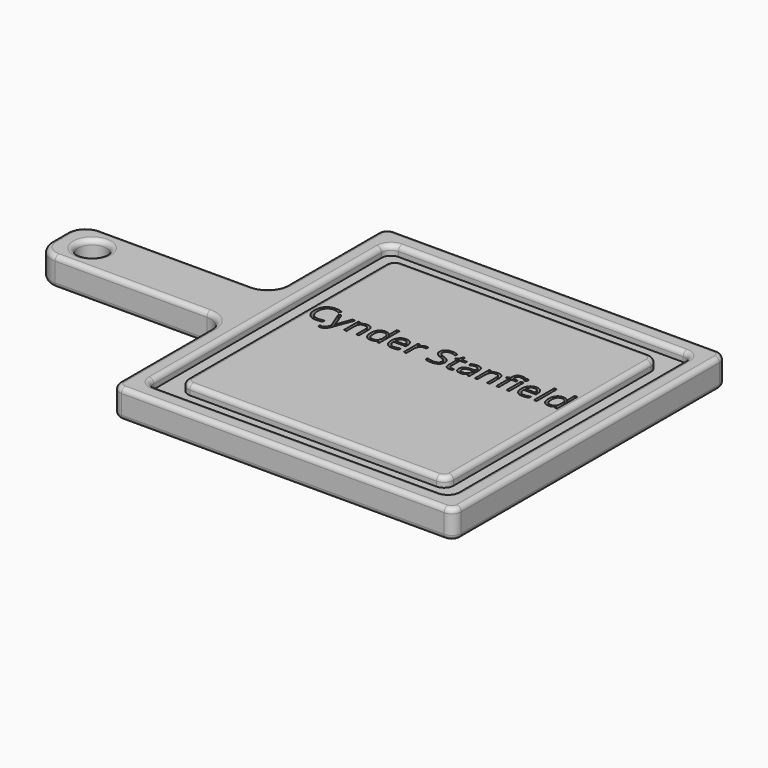
from build123d import *

# Parameters (mm, degrees)
F0_W          = 127
F0_H          = 38.1
F1_DEPTH      = 19.05
F2_R          = 9.525
F3_DEPTH      = 25.4
F5_DEPTH      = 6.35
F6_R          = 6.35
F7_R          = 6.35
F8_R          = 12.7
F9_R          = 3.175
F10_TEXT_SIZE = 22.3825058862
F11_DEPTH     = 5.08


# Not quite as in the source:
# - Text() gives the source's letters only with a copy of the font that has no kerning and outlines rounded to 1/6400 em; it was checked with that copy


with BuildPart() as f1:
    # F0 (on Top) → F1 (new body)
    with BuildSketch(Plane.XY):
        Polygon((0, 95.25), (0, 0), (228.6, 0), (228.6, 228.6), (0, 228.6), (0, 133.35), align=None)
        with Locations((-63.5, 114.3)):
            Rectangle(F0_W, F0_H)
    extrude(amount=F1_DEPTH)

    # F2 (on face) → F3 (cut)
    with BuildSketch(Plane.XY.offset(19.05)):
        with Locations((-104.775, 114.3)):
            Circle(F2_R)
    extrude(amount=-F3_DEPTH, mode=Mode.SUBTRACT)

    # F4 (on face) → F5 (cut)
    with BuildSketch(Plane.XY.offset(19.05)):
        Polygon((12.6999960899, 95.25), (12.6999960899, 12.6999960899), (215.9000039101, 12.6999960899), (215.9000039101, 215.9000039101), (12.6999960899, 215.9000039101), (12.6999960899, 133.35), align=None)
        Polygon((25.4000024557, 95.25), (25.4000024557, 133.35), (25.4000024557, 203.1999975443), (203.1999975443, 203.1999975443), (203.1999975443, 25.4000024557), (25.4000024557, 25.4000024557), align=None, mode=Mode.SUBTRACT)
    extrude(amount=-F5_DEPTH, mode=Mode.SUBTRACT)

    # F6
    f6_edges = [f1.edges().sort_by_distance(p)[0] for p in [
        (12.699996, 215.900004, 15.875),
        (12.699996, 12.699996, 15.875),
        (215.900004, 12.699996, 15.875),
        (215.900004, 215.900004, 15.875),
        (25.400002, 203.199998, 15.875),
        (203.199998, 203.199998, 15.875),
        (203.199998, 25.400002, 15.875),
        (25.400002, 25.400002, 15.875),
    ]]
    fillet(f6_edges, radius=F6_R)

    # F7
    f7_edges = [f1.edges().sort_by_distance(p)[0] for p in [
        (0, 0, 9.525),
        (228.6, 0, 9.525),
        (228.6, 228.6, 9.525),
        (0, 228.6, 9.525),
    ]]
    fillet(f7_edges, radius=F7_R)

    # F8
    f8_edges = [f1.edges().sort_by_distance(p)[0] for p in [
        (0, 133.35, 9.525),
        (0, 95.25, 9.525),
        (-127, 95.25, 9.525),
        (-127, 133.35, 9.525),
    ]]
    fillet(f8_edges, radius=F8_R)

    # F9
    f9_edges = [f1.edges().sort_by_distance(p)[0] for p in [
        (0, 44.45, 19.05),
        (-3.719744, 91.530256, 19.05),
        (1.859872, 1.859872, 19.05),
        (-63.5, 95.25, 19.05),
        (114.3, 0, 19.05),
        (-123.280256, 98.969744, 19.05),
        (226.740128, 1.859872, 19.05),
        (-127, 114.3, 19.05),
        (228.6, 114.3, 19.05),
        (-123.280256, 129.630256, 19.05),
        (226.740128, 226.740128, 19.05),
        (-63.5, 133.35, 19.05),
        (114.3, 228.6, 19.05),
        (-3.719744, 137.069744, 19.05),
        (1.859872, 226.740128, 19.05),
        (0, 184.15, 19.05),
        (114.3, 12.699996, 19.05),
        (14.559868, 14.559868, 19.05),
        (214.040132, 14.559868, 19.05),
        (12.699996, 114.3, 19.05),
        (215.900004, 114.3, 19.05),
        (14.559868, 214.040132, 19.05),
        (214.040132, 214.040132, 19.05),
        (114.3, 215.900004, 19.05),
        (-114.3, 114.3, 19.05),
        (114.3, 203.199998, 19.05),
        (27.259874, 201.340126, 19.05),
        (201.340126, 201.340126, 19.05),
        (25.400002, 114.3, 19.05),
        (203.199998, 114.3, 19.05),
        (27.259874, 27.259874, 19.05),
        (201.340126, 27.259874, 19.05),
        (114.3, 25.400002, 19.05),
        (0, 44.45, 0),
        (-3.719744, 91.530256, 0),
        (1.859872, 1.859872, 0),
        (-63.5, 95.25, 0),
        (114.3, 0, 0),
        (-123.280256, 98.969744, 0),
        (226.740128, 1.859872, 0),
        (-127, 114.3, 0),
        (228.6, 114.3, 0),
        (-123.280256, 129.630256, 0),
        (226.740128, 226.740128, 0),
        (-63.5, 133.35, 0),
        (114.3, 228.6, 0),
        (-3.719744, 137.069744, 0),
        (1.859872, 226.740128, 0),
        (0, 184.15, 0),
        (-114.3, 114.3, 0),
    ]]
    fillet(f9_edges, radius=F9_R)

    # F10 (on face) → F11 (cut)
    with BuildSketch(Plane.XY.offset(19.05)):
        with Locations((28.5750024557, 124.0698920125)):
            Text('Cynder Stanfield', F10_TEXT_SIZE, font='Open Sans', text_align=(TextAlign.LEFT, TextAlign.BOTTOM))
    extrude(amount=-F11_DEPTH, mode=Mode.SUBTRACT)


solid = f1.part
